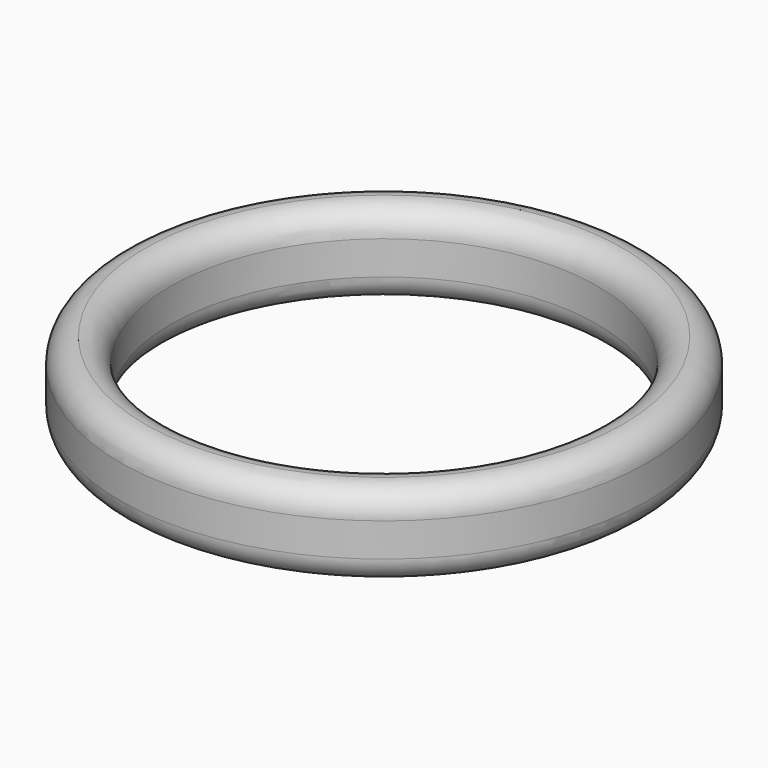
from build123d import *

# Parameters (mm, degrees)
F0_R     = 15.7
F0_R_2   = 12.7
F1_DEPTH = 5
F2_R     = 1.49999


# Not quite as in the source:
# - a fillet or chamfer is up to 0.001 mm smaller than in the source, because OpenCascade refuses the exact size


with BuildPart() as f1:
    # F0 (on Top) → F1 (new body)
    with BuildSketch(Plane.XY):
        Circle(F0_R)
        Circle(F0_R_2, mode=Mode.SUBTRACT)
    extrude(amount=F1_DEPTH)

    # F2 (radius 1.5 in the source; OpenCascade refuses exactly that, so slightly less here)
    f2_edges = [f1.edges().sort_by_distance(p)[0] for p in [
        (-15.7, 0, 5),
        (-12.7, 0, 5),
        (-15.7, 0, 0),
        (-12.7, 0, 0),
    ]]
    fillet(f2_edges, radius=F2_R)


solid = f1.part
